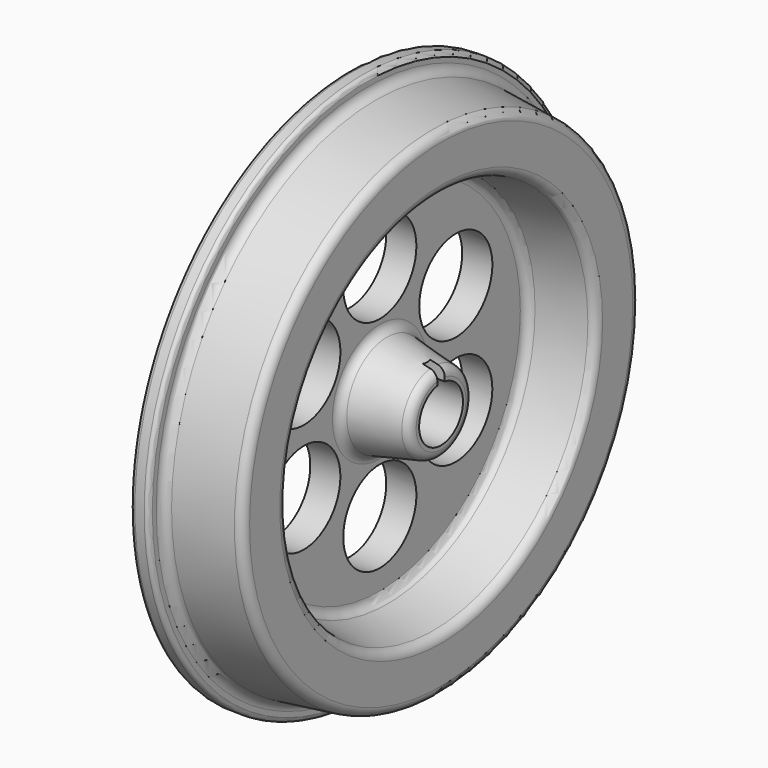
from build123d import *

# Parameters (mm, degrees)
F2_R            = 15
F3_DEPTH        = 50
F4_R            = 25
F5_DEPTH        = 16.491995675
F5_COPIES_COUNT = 6
F6_R            = 17.5
F7_DEPTH        = 5
F8_R            = 5
F9_R            = 2.5
F10_W           = 5
F10_H           = 9.5783152908
F11_DEPTH       = 50.0010001


# Not quite as in the source:
# - a pattern or mirror of a feature is missing from the dataset's text; its kind, count and spacing are read off the source's solid


with BuildPart() as f1:
    # F0 (on Top) → F1 (revolve)
    with BuildSketch(Plane.XY):
        Polygon((0, 150), (0, 0), (50, 0), (50, 21.0459418595), (16.491995675, 28.3900303053), (16.491995675, 100.2885912763), (50.0555746781, 106.2067558237), (50.0555746781, 135.4332249232), (10, 140.3514310718), (10, 150), align=None)
    revolve(axis=Axis((25, 0, 0), (-1, 0, 0)))

    # F2 (on face) → F3 (cut, through all)
    with BuildSketch(Plane.YZ.offset(50)):
        Circle(F2_R)
    extrude(amount=-F3_DEPTH, mode=Mode.SUBTRACT)

    # F4 (on face) → F5 (cut, through all)
    with BuildSketch(Plane.YZ.offset(16.491995675)):
        with Locations((0, 60)):
            Circle(F4_R)
    f5 = extrude(amount=-F5_DEPTH, mode=Mode.SUBTRACT)

    # F5_copies: F5 ×6 about axis
    f5_copies_axis = Axis((0, 0, 0), (1, 0, 0))
    for i in range(1, F5_COPIES_COUNT):
        add(f5.rotate(f5_copies_axis, i * 360 / F5_COPIES_COUNT), mode=Mode.SUBTRACT)

    # F6 (on face) → F7 (cut)
    with BuildSketch(Plane(origin=(0, 0, 0), x_dir=(0, -1, 0), z_dir=(-1, 0, 0))):
        Circle(F6_R)
    extrude(amount=-F7_DEPTH, mode=Mode.SUBTRACT)

    # F8
    f8_edges = [f1.edges().sort_by_distance(p)[0] for p in [
        (16.491996, -100.288591, 0),
        (50.055575, -106.206756, 0),
        (50.055575, -135.433225, 0),
        (10, -140.351431, 0),
        (50, -21.045942, 0),
        (16.491996, -28.39003, 0),
    ]]
    fillet(f8_edges, radius=F8_R)

    # F9
    f9_edges = [f1.edges().sort_by_distance(p)[0] for p in [
        (10, -150, 0),
        (0, -150, 0),
    ]]
    fillet(f9_edges, radius=F9_R)

    # F10 (on face) → F11 (cut, through all)
    with BuildSketch(Plane(origin=(0, 0, 0), x_dir=(0, -1, 0), z_dir=(-1, 0, 0))):
        with Locations((0, 17.8858903802)):
            Rectangle(F10_W, F10_H)
    extrude(amount=-F11_DEPTH, mode=Mode.SUBTRACT)


solid = f1.part
